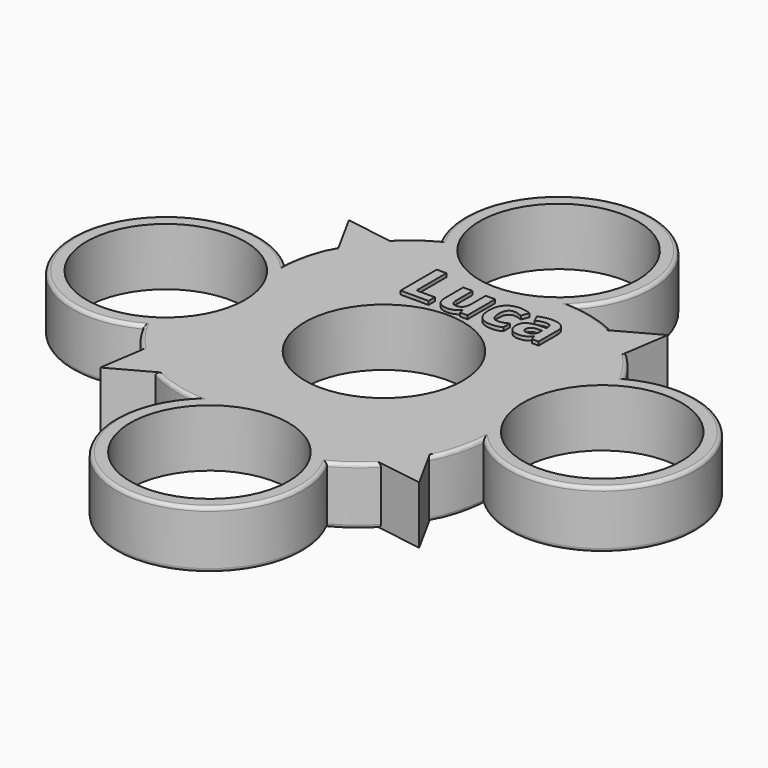
from build123d import *

# Parameters (mm, degrees)
F0_R         = 11
F1_DEPTH     = 8
F2_R         = 0.5
F4_TEXT_SIZE = 8.8205651587
F5_DEPTH     = 0.5


# Not quite as in the source:
# - Text() gives the source's letters only with a copy of the font that has no kerning and outlines rounded to 1/6400 em; it was checked with that copy


with BuildPart() as f1:
    # F0 (on Top) → F1 (new body)
    with BuildSketch(Plane.XY):
        with BuildLine():
            ThreePointArc((16.3477687761, 19.3002136583), (12.9484463268, 20.6437071995), (9.3520145888, 21.2964297773))
            ThreePointArc((9.3520145888, 21.2964297773), (1.8306831083, 43.1968246623), (-11.4989804127, 24.2622585523))
            ThreePointArc((-11.4989804127, 24.2622585523), (-13.9695826758, 22.6853162416), (-16.161771108, 20.7398259509))
            Line((-16.161771108, 20.7398259509), (-22.2147591412, 21.6616932303))
            Line((-22.2147591412, 21.6616932303), (-19.3002136583, 16.3477687761))
            ThreePointArc((-19.3002136583, 16.3477687761), (-20.6437071995, 12.9484463268), (-21.2964297773, 9.3520145888))
            ThreePointArc((-21.2964297773, 9.3520145888), (-43.1968246623, 1.8306831083), (-24.2622585523, -11.4989804127))
            ThreePointArc((-24.2622585523, -11.4989804127), (-22.6853162416, -13.9695826758), (-20.7398259509, -16.161771108))
            Line((-20.7398259509, -16.161771108), (-21.6616932303, -22.2147591412))
            Line((-21.6616932303, -22.2147591412), (-16.3477687761, -19.3002136583))
            ThreePointArc((-16.3477687761, -19.3002136583), (-12.9484463268, -20.6437071995), (-9.3520145888, -21.2964297773))
            ThreePointArc((-9.3520145888, -21.2964297773), (-1.8306831083, -43.1968246623), (11.4989804127, -24.2622585523))
            ThreePointArc((11.4989804127, -24.2622585523), (13.9695826758, -22.6853162416), (16.161771108, -20.7398259509))
            Line((16.161771108, -20.7398259509), (22.2147591412, -21.6616932303))
            Line((22.2147591412, -21.6616932303), (19.3002136583, -16.3477687761))
            ThreePointArc((19.3002136583, -16.3477687761), (20.6437071995, -12.9484463268), (21.2964297773, -9.3520145888))
            ThreePointArc((21.2964297773, -9.3520145888), (43.1968246623, -1.8306831083), (24.2622585523, 11.4989804127))
            ThreePointArc((24.2622585523, 11.4989804127), (22.6853162416, 13.9695826758), (20.7398259509, 16.161771108))
            Line((20.7398259509, 16.161771108), (21.6616932303, 22.2147591412))
            Line((21.6616932303, 22.2147591412), (16.3477687761, 19.3002136583))
        make_face()
        with Locations((0, -30.3263701499)):
            Circle(F0_R, mode=Mode.SUBTRACT)
        with Locations((-30.3263701499, 0)):
            Circle(F0_R, mode=Mode.SUBTRACT)
        Circle(F0_R, mode=Mode.SUBTRACT)
        with Locations((30.3263701499, 0)):
            Circle(F0_R, mode=Mode.SUBTRACT)
        with Locations((0, 30.3263701499)):
            Circle(F0_R, mode=Mode.SUBTRACT)
    extrude(amount=F1_DEPTH)

    # F2
    f2_edges = [f1.edges().sort_by_distance(p)[0] for p in [
        (-20.643707, 12.948446, 8),
        (-20.643707, 12.948446, 0),
        (20.643707, -12.948446, 8),
        (20.643707, -12.948446, 0),
        (13.969583, -22.685316, 0),
        (13.969583, -22.685316, 8),
        (-12.948446, -20.643707, 8),
        (-12.948446, -20.643707, 0),
        (-22.685316, -13.969583, 0),
        (-22.685316, -13.969583, 8),
        (-13.969583, 22.685316, 8),
        (-13.969583, 22.685316, 0),
        (12.948446, 20.643707, 0),
        (12.948446, 20.643707, 8),
        (22.685316, 13.969583, 8),
        (22.685316, 13.969583, 0),
        (43.196825, -1.830683, 8),
        (43.196825, -1.830683, 0),
        (1.830683, 43.196825, 0),
        (1.830683, 43.196825, 8),
        (-1.830683, -43.196825, 8),
        (-1.830683, -43.196825, 0),
        (-43.196825, 1.830683, 8),
        (-43.196825, 1.830683, 0),
    ]]
    fillet(f2_edges, radius=F2_R)


with BuildPart() as f5:
    # F4 (on offset) → F5 (new body)
    with BuildSketch(Plane.XY.offset(8)):
        with Locations((-7.7116941102, 11.5221785381)):
            Text('Luca', F4_TEXT_SIZE, font='Open Sans', font_style=FontStyle.BOLD, text_align=(TextAlign.LEFT, TextAlign.BOTTOM))
    extrude(amount=F5_DEPTH)


solid = Compound([f1.part, f5.part])
